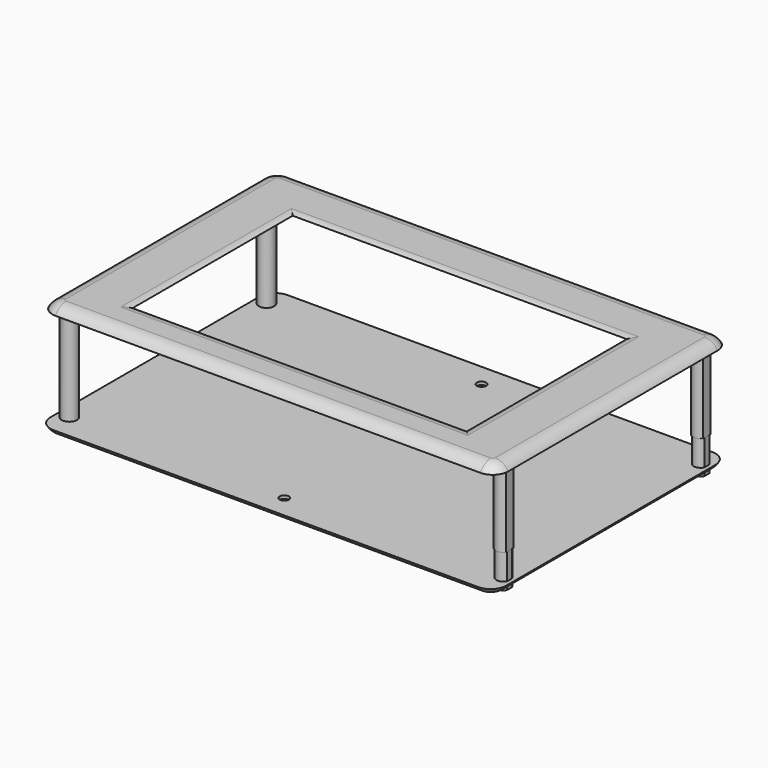
from build123d import *

# Parameters (mm, degrees)
F0_W          = 134
F0_H          = 95
F0_R          = 3
F0_W_2        = 120
F0_H_2        = 76
F0_W_3        = 116.5
F0_H_3        = 70.5
F0_W_4        = 108.5
F0_H_4        = 65
F0_R_2        = 1.5
F1_DEPTH      = 2.5
F2_DEPTH      = 2
F3_DEPTH      = 0.5
F4_T1_DEPTH   = 108.5
F4_T3_DEPTH   = 65
F4_T5_DEPTH   = 85
F4_T7_DEPTH   = 138
F4_T10_ANGLE  = 90
F4_T12_ANGLE  = 90
F4_T14_ANGLE  = 90
F4_T16_ANGLE  = 90
F4_T21_DEPTH  = 70.4491776016
F4_T25_DEPTH  = 113.9491776016
F4_T32_DEPTH  = 70.4491776016
F4_T36_DEPTH  = 113.9491776016
F4_T43_DEPTH  = 113.9491776016
F4_T47_DEPTH  = 70.4491776016
F4_T54_DEPTH  = 70.4491776016
F4_T58_DEPTH  = 113.9491776016
F5_DEPTH      = 35
F6_DEPTH      = 24
F8_R          = 2.5
F8_R_2        = 1.5
F9_DEPTH      = 2.5
F10_T1_DEPTH  = 85
F10_T3_DEPTH  = 138
F10_T6_ANGLE  = 90
F10_T8_ANGLE  = 90
F10_T10_ANGLE = 90
F10_T12_ANGLE = 90
F11_DEPTH     = 1.5
F13_R         = 1.75
F14_DEPTH     = 11


# Not quite as in the source:
# - a fillet or chamfer that OpenCascade refuses, or shapes differently, is made with other operations: its cross-section is extruded or revolved along the edge and cut away or added


with BuildPart() as f1:
    # F0 (on Top) → F1 (new body)
    with BuildSketch(Plane.XY):
        with Locations((0.2218604458, 0.5862068966)):
            Rectangle(F0_W, F0_H)
        with Locations((-57.2781395542, -41.4137931034)):
            Circle(F0_R, mode=Mode.SUBTRACT)
        with Locations((57.7218604458, -41.4137931034)):
            Circle(F0_R, mode=Mode.SUBTRACT)
        with Locations((0.2218604458, 0.0862068966)):
            Rectangle(F0_W_2, F0_H_2, mode=Mode.SUBTRACT)
        with Locations((-57.2781395542, 42.5862068966)):
            Circle(F0_R, mode=Mode.SUBTRACT)
        with Locations((57.7218604458, 42.5862068966)):
            Circle(F0_R, mode=Mode.SUBTRACT)
        with BuildLine():
            Line((-66.7781395542, -46.9137931034), (-66.7781395542, 48.0862068966))
            Line((-66.7781395542, 48.0862068966), (-68.7781395542, 48.0862068966))
            ThreePointArc((-68.7781395542, 48.0862068966), (-72.3136734602, 46.6217408025), (-73.7781395542, 43.0862068966))
            Line((-73.7781395542, 43.0862068966), (-73.7781395542, -41.9137931034))
            ThreePointArc((-73.7781395542, -41.9137931034), (-72.3136734602, -45.4493270094), (-68.7781395542, -46.9137931034))
            Line((-68.7781395542, -46.9137931034), (-66.7781395542, -46.9137931034))
        make_face()
        with BuildLine():
            ThreePointArc((-72.2781395542, -37.9473820925), (-67.7781395542, -39.4473820925), (-72.2781395542, -40.9473820925))
            Line((-72.2781395542, -40.9473820925), (-72.2781395542, -37.9473820925))
        make_face(mode=Mode.SUBTRACT)
        with BuildLine():
            ThreePointArc((-72.2781395542, 42.0910126865), (-67.7781395542, 40.5910126865), (-72.2781395542, 39.0910126865))
            Line((-72.2781395542, 39.0910126865), (-72.2781395542, 42.0910126865))
        make_face(mode=Mode.SUBTRACT)
        with BuildLine():
            Line((69.2218604458, 48.0862068966), (67.2218604458, 48.0862068966))
            Line((67.2218604458, 48.0862068966), (67.2218604458, -46.9137931034))
            Line((67.2218604458, -46.9137931034), (69.2218604458, -46.9137931034))
            ThreePointArc((69.2218604458, -46.9137931034), (72.7573943517, -45.4493270094), (74.2218604458, -41.9137931034))
            Line((74.2218604458, -41.9137931034), (74.2218604458, 43.0862068966))
            ThreePointArc((74.2218604458, 43.0862068966), (72.7573943517, 46.6217408025), (69.2218604458, 48.0862068966))
        make_face()
        with BuildLine():
            ThreePointArc((72.7218604458, -40.9469694146), (68.2218604458, -39.4469694146), (72.7218604458, -37.9469694146))
            Line((72.7218604458, -37.9469694146), (72.7218604458, -40.9469694146))
        make_face(mode=Mode.SUBTRACT)
        with BuildLine():
            ThreePointArc((72.7218604458, 39.0908259189), (68.2218604458, 40.5908259189), (72.7218604458, 42.0908259189))
            Line((72.7218604458, 42.0908259189), (72.7218604458, 39.0908259189))
        make_face(mode=Mode.SUBTRACT)
        with Locations((-57.2781395542, 42.5862068966)):
            Circle(F0_R)
        with Locations((57.7218604458, 42.5862068966)):
            Circle(F0_R)
        with Locations((57.7218604458, -41.4137931034)):
            Circle(F0_R)
        with Locations((-57.2781395542, -41.4137931034)):
            Circle(F0_R)
        with Locations((0.2218604458, 0.0862068966)):
            Rectangle(F0_W_2, F0_H_2)
        with Locations((0.4718604458, -1.1637931034)):
            Rectangle(F0_W_3, F0_H_3, mode=Mode.SUBTRACT)
        with Locations((0.4718604458, -1.1637931034)):
            Rectangle(F0_W_3, F0_H_3)
        with Locations((0.4718604458, -1.9137931034)):
            Rectangle(F0_W_4, F0_H_4, mode=Mode.SUBTRACT)
        with BuildLine():
            Line((-72.2781395542, 42.0910126865), (-72.2781395542, 39.0910126865))
            ThreePointArc((-72.2781395542, 39.0910126865), (-67.7781395542, 40.5910126865), (-72.2781395542, 42.0910126865))
        make_face()
        with Locations((-70.2781395542, 40.5910126865)):
            Circle(F0_R_2, mode=Mode.SUBTRACT)
        with Locations((-70.2781395542, 40.5910126865)):
            Circle(F0_R_2)
        with BuildLine():
            Line((-72.2781395542, -37.9473820925), (-72.2781395542, -40.9473820925))
            ThreePointArc((-72.2781395542, -40.9473820925), (-67.7781395542, -39.4473820925), (-72.2781395542, -37.9473820925))
        make_face()
        with Locations((-70.2781395542, -39.4473820925)):
            Circle(F0_R_2, mode=Mode.SUBTRACT)
        with Locations((-70.2781395542, -39.4473820925)):
            Circle(F0_R_2)
        with BuildLine():
            Line((72.7218604458, -40.9469694146), (72.7218604458, -37.9469694146))
            ThreePointArc((72.7218604458, -37.9469694146), (68.2218604458, -39.4469694146), (72.7218604458, -40.9469694146))
        make_face()
        with Locations((70.7218604458, -39.4469694146)):
            Circle(F0_R_2, mode=Mode.SUBTRACT)
        with Locations((70.7218604458, -39.4469694146)):
            Circle(F0_R_2)
        with BuildLine():
            Line((72.7218604458, 39.0908259189), (72.7218604458, 42.0908259189))
            ThreePointArc((72.7218604458, 42.0908259189), (68.2218604458, 40.5908259189), (72.7218604458, 39.0908259189))
        make_face()
        with Locations((70.7218604458, 40.5908259189)):
            Circle(F0_R_2, mode=Mode.SUBTRACT)
        with Locations((70.7218604458, 40.5908259189)):
            Circle(F0_R_2)
    extrude(amount=F1_DEPTH)

    # F0 (on Top) → F2 (cut)
    with BuildSketch(Plane.XY):
        with Locations((-57.2781395542, 42.5862068966)):
            Circle(F0_R)
        with Locations((-57.2781395542, -41.4137931034)):
            Circle(F0_R)
        with Locations((57.7218604458, -41.4137931034)):
            Circle(F0_R)
        with Locations((57.7218604458, 42.5862068966)):
            Circle(F0_R)
        with Locations((0.4718604458, -1.1637931034)):
            Rectangle(F0_W_3, F0_H_3)
        with Locations((0.4718604458, -1.9137931034)):
            Rectangle(F0_W_4, F0_H_4, mode=Mode.SUBTRACT)
    extrude(amount=F2_DEPTH, mode=Mode.SUBTRACT)

    # F0 (on Top) → F3 (cut)
    with BuildSketch(Plane.XY):
        with Locations((0.2218604458, 0.0862068966)):
            Rectangle(F0_W_2, F0_H_2)
        with Locations((0.4718604458, -1.1637931034)):
            Rectangle(F0_W_3, F0_H_3, mode=Mode.SUBTRACT)
    extrude(amount=F3_DEPTH, mode=Mode.SUBTRACT)

    # F4: fillet of radius 5 on 12 edges, made by hand

    # F4_s2 → F4_t1 (cut)
    with BuildSketch(Plane.YZ.offset(-53.7781395542)):
        with BuildLine():
            ThreePointArc((32.7658779005, 2.5004), (31.647646516, 2.3737873637), (30.5860325565, 2.0003600077))
            Line((30.5860325565, 2.0003600077), (30.3680480221, 2.450492577))
            ThreePointArc((30.3680480221, 2.450492577), (30.086070328, 2.2501800039), (30.086070328, 2.5))
            Line((30.086070328, 2.5), (30.5862068966, 3.0001365685))
            ThreePointArc((30.5862068966, 3.0001365685), (31.6760423985, 3.0001365685), (32.7658779005, 3.0005365685))
            Line((32.7658779005, 3.0005365685), (32.7658779005, 2.5004))
        make_face()
        with BuildLine():
            ThreePointArc((-36.5934641074, 2.5004), (-35.4752327229, 2.3737873637), (-34.4136187634, 2.0003600077))
            Line((-34.4136187634, 2.0003600077), (-34.195634229, 2.450492577))
            ThreePointArc((-34.195634229, 2.450492577), (-33.9136565349, 2.2501800039), (-33.9136565349, 2.5))
            Line((-33.9136565349, 2.5), (-34.4137931034, 3.0001365685))
            ThreePointArc((-34.4137931034, 3.0001365685), (-35.5036286054, 3.0001365685), (-36.5934641074, 3.0005365685))
            Line((-36.5934641074, 3.0005365685), (-36.5934641074, 2.5004))
        make_face()
    extrude(amount=F4_T1_DEPTH, mode=Mode.SUBTRACT)

    # F4_s4 → F4_t3 (cut)
    with BuildSketch(Plane.XZ.offset(-30.5862068966)):
        with BuildLine():
            ThreePointArc((-55.9578105582, 2.5004), (-54.8395791736, 2.3737873637), (-53.7779652142, 2.0003600077))
            Line((-53.7779652142, 2.0003600077), (-53.5599806798, 2.450492577))
            ThreePointArc((-53.5599806798, 2.450492577), (-53.2780029857, 2.2501800039), (-53.2780029857, 2.5))
            Line((-53.2780029857, 2.5), (-53.7781395542, 3.0001365685))
            ThreePointArc((-53.7781395542, 3.0001365685), (-54.8679750562, 3.0001365685), (-55.9578105582, 3.0005365685))
            Line((-55.9578105582, 3.0005365685), (-55.9578105582, 2.5004))
        make_face()
        with BuildLine():
            ThreePointArc((56.9015314497, 2.5004), (55.7833000652, 2.3737873637), (54.7216861058, 2.0003600077))
            Line((54.7216861058, 2.0003600077), (54.5037015714, 2.450492577))
            ThreePointArc((54.5037015714, 2.450492577), (54.2217238772, 2.2501800039), (54.2217238772, 2.5))
            Line((54.2217238772, 2.5), (54.7218604458, 3.0001365685))
            ThreePointArc((54.7218604458, 3.0001365685), (55.8116959477, 3.0001365685), (56.9015314497, 3.0005365685))
            Line((56.9015314497, 3.0005365685), (56.9015314497, 2.5004))
        make_face()
    extrude(amount=F4_T3_DEPTH, mode=Mode.SUBTRACT)

    # F4_s6 → F4_t5 (cut)
    with BuildSketch(Plane.XZ.offset(-43.0862068966)):
        with BuildLine():
            ThreePointArc((69.891175924, 2.5004), (72.3916173144, 1.8304834454), (74.2222068336, 0.0002000386))
            Line((74.2222068336, 0.0002000386), (74.6553099246, 0.250316611))
            ThreePointArc((74.6553099246, 0.250316611), (74.7219970143, 1.2501000193), (74.7219970143, 2.5))
            Line((74.7219970143, 2.5), (74.2218604458, 3.0001365685))
            ThreePointArc((74.2218604458, 3.0001365685), (72.0565181849, 3.0001365685), (69.891175924, 3.0005365685))
            Line((69.891175924, 3.0005365685), (69.891175924, 2.5004))
        make_face()
        with BuildLine():
            ThreePointArc((-73.7784859421, 0.0002000386), (-71.9478964228, 1.8304834454), (-69.4474550324, 2.5004))
            Line((-69.4474550324, 2.5004), (-69.4474550324, 3.0005365685))
            ThreePointArc((-69.4474550324, 3.0005365685), (-71.6127972933, 3.0001365685), (-73.7781395542, 3.0001365685))
            Line((-73.7781395542, 3.0001365685), (-74.2782761228, 2.5))
            ThreePointArc((-74.2782761228, 2.5), (-74.2782761228, 1.2501000193), (-74.211589033, 0.250316611))
            Line((-74.211589033, 0.250316611), (-73.7784859421, 0.0002000386))
        make_face()
    extrude(amount=F4_T5_DEPTH, mode=Mode.SUBTRACT)

    # F4_s8 → F4_t7 (cut)
    with BuildSketch(Plane.YZ.offset(-68.7781395542)):
        with BuildLine():
            ThreePointArc((48.0865532844, 0.0002000386), (46.2559637652, 1.8304834454), (43.7555223748, 2.5004))
            Line((43.7555223748, 2.5004), (43.7555223748, 3.0005365685))
            ThreePointArc((43.7555223748, 3.0005365685), (45.9208646357, 3.0001365685), (48.0862068966, 3.0001365685))
            Line((48.0862068966, 3.0001365685), (48.5863434651, 2.5))
            ThreePointArc((48.5863434651, 2.5), (48.5863434651, 1.2501000193), (48.5196563754, 0.250316611))
            Line((48.5196563754, 0.250316611), (48.0865532844, 0.0002000386))
        make_face()
        with BuildLine():
            ThreePointArc((-42.5831085817, 2.5004), (-45.0835499721, 1.8304834454), (-46.9141394913, 0.0002000386))
            Line((-46.9141394913, 0.0002000386), (-47.3472425823, 0.250316611))
            ThreePointArc((-47.3472425823, 0.250316611), (-47.413929672, 1.2501000193), (-47.413929672, 2.5))
            Line((-47.413929672, 2.5), (-46.9137931034, 3.0001365685))
            ThreePointArc((-46.9137931034, 3.0001365685), (-44.7484508426, 3.0001365685), (-42.5831085817, 3.0005365685))
            Line((-42.5831085817, 3.0005365685), (-42.5831085817, 2.5004))
        make_face()
    extrude(amount=F4_T7_DEPTH, mode=Mode.SUBTRACT)

    # F4_s9 → F4_t10 (revolve, cut)
    with BuildSketch(Plane.XZ.offset(-43.0862068966)):
        with BuildLine():
            ThreePointArc((69.891175924, 2.5004), (72.3916173144, 1.8304834454), (74.2222068336, 0.0002000386))
            Line((74.2222068336, 0.0002000386), (74.6553099246, 0.250316611))
            ThreePointArc((74.6553099246, 0.250316611), (74.7219970143, 1.2501000193), (74.7219970143, 2.5))
            Line((74.7219970143, 2.5), (74.2218604458, 3.0001365685))
            ThreePointArc((74.2218604458, 3.0001365685), (72.0565181849, 3.0001365685), (69.891175924, 3.0005365685))
            Line((69.891175924, 3.0005365685), (69.891175924, 2.5004))
        make_face()
    revolve(axis=Axis((69.2218604458, 43.0862068966, 2.5), (0, 0, 1)), revolution_arc=F4_T10_ANGLE, mode=Mode.SUBTRACT)

    # F4_s11 → F4_t12 (revolve, cut)
    with BuildSketch(Plane.YZ.offset(69.2218604458)):
        with BuildLine():
            ThreePointArc((-42.5831085817, 2.5004), (-45.0835499721, 1.8304834454), (-46.9141394913, 0.0002000386))
            Line((-46.9141394913, 0.0002000386), (-47.3472425823, 0.250316611))
            ThreePointArc((-47.3472425823, 0.250316611), (-47.413929672, 1.2501000193), (-47.413929672, 2.5))
            Line((-47.413929672, 2.5), (-46.9137931034, 3.0001365685))
            ThreePointArc((-46.9137931034, 3.0001365685), (-44.7484508426, 3.0001365685), (-42.5831085817, 3.0005365685))
            Line((-42.5831085817, 3.0005365685), (-42.5831085817, 2.5004))
        make_face()
    revolve(axis=Axis((69.2218604458, -41.9137931034, 2.5), (0, 0, 1)), revolution_arc=F4_T12_ANGLE, mode=Mode.SUBTRACT)

    # F4_s13 → F4_t14 (revolve, cut)
    with BuildSketch(Plane.XZ.offset(41.9137931034)):
        with BuildLine():
            ThreePointArc((-69.4474550324, 2.5004), (-71.9478964228, 1.8304834454), (-73.7784859421, 0.0002000386))
            Line((-73.7784859421, 0.0002000386), (-74.211589033, 0.250316611))
            ThreePointArc((-74.211589033, 0.250316611), (-74.2782761228, 1.2501000193), (-74.2782761228, 2.5))
            Line((-74.2782761228, 2.5), (-73.7781395542, 3.0001365685))
            ThreePointArc((-73.7781395542, 3.0001365685), (-71.6127972933, 3.0001365685), (-69.4474550324, 3.0005365685))
            Line((-69.4474550324, 3.0005365685), (-69.4474550324, 2.5004))
        make_face()
    revolve(axis=Axis((-68.7781395542, -41.9137931034, 2.5), (0, 0, 1)), revolution_arc=F4_T14_ANGLE, mode=Mode.SUBTRACT)

    # F4_s15 → F4_t16 (revolve, cut)
    with BuildSketch(Plane.YZ.offset(-68.7781395542)):
        with BuildLine():
            ThreePointArc((48.0865532844, 0.0002000386), (46.2559637652, 1.8304834454), (43.7555223748, 2.5004))
            Line((43.7555223748, 2.5004), (43.7555223748, 3.0005365685))
            ThreePointArc((43.7555223748, 3.0005365685), (45.9208646357, 3.0001365685), (48.0862068966, 3.0001365685))
            Line((48.0862068966, 3.0001365685), (48.5863434651, 2.5))
            ThreePointArc((48.5863434651, 2.5), (48.5863434651, 1.2501000193), (48.5196563754, 0.250316611))
            Line((48.5196563754, 0.250316611), (48.0865532844, 0.0002000386))
        make_face()
    revolve(axis=Axis((-68.7781395542, 43.0862068966, 2.5), (0, 0, 1)), revolution_arc=F4_T16_ANGLE, mode=Mode.SUBTRACT)


with BuildPart() as f4_tool19:
    # F4_s20 → F4_t21 (new body)
    with BuildSketch(Plane.XZ.offset(34.4137931034)):
        with BuildLine():
            ThreePointArc((-55.9578105582, 2.5004), (-54.8395791736, 2.3737873637), (-53.7779652142, 2.0003600077))
            Line((-53.7779652142, 2.0003600077), (-53.5599806798, 2.450492577))
            ThreePointArc((-53.5599806798, 2.450492577), (-53.2780029857, 2.2501800039), (-53.2780029857, 2.5))
            Line((-53.2780029857, 2.5), (-53.7781395542, 3.0001365685))
            ThreePointArc((-53.7781395542, 3.0001365685), (-54.8679750562, 3.0001365685), (-55.9578105582, 3.0005365685))
            Line((-55.9578105582, 3.0005365685), (-55.9578105582, 2.5004))
        make_face()
    extrude(amount=-F4_T21_DEPTH)

    split(bisect_by=Plane.XZ.offset(-30.5862068966), keep=Keep.BOTTOM)


with BuildPart() as f4_tool23:
    # F4_s24 → F4_t25 (new body)
    with BuildSketch(Plane.YZ.offset(-59.2273171558)):
        with BuildLine():
            ThreePointArc((32.7658779005, 2.5004), (31.647646516, 2.3737873637), (30.5860325565, 2.0003600077))
            Line((30.5860325565, 2.0003600077), (30.3680480221, 2.450492577))
            ThreePointArc((30.3680480221, 2.450492577), (30.086070328, 2.2501800039), (30.086070328, 2.5))
            Line((30.086070328, 2.5), (30.5862068966, 3.0001365685))
            ThreePointArc((30.5862068966, 3.0001365685), (31.6760423985, 3.0001365685), (32.7658779005, 3.0005365685))
            Line((32.7658779005, 3.0005365685), (32.7658779005, 2.5004))
        make_face()
    extrude(amount=F4_T25_DEPTH)

    split(bisect_by=Plane.YZ.offset(-53.7781395542), keep=Keep.BOTTOM)


with BuildPart() as f4_tool19_1:
    add(f4_tool19.part)

    # F4_t27: intersect F4_tool23
    add(f4_tool23.part, mode=Mode.INTERSECT)


with BuildPart() as f1_1:
    add(f1.part)

    # F4_t17: cut F4_tool19
    add(f4_tool19_1.part, mode=Mode.SUBTRACT)


with BuildPart() as f4_tool30:
    # F4_s31 → F4_t32 (new body)
    with BuildSketch(Plane.XZ.offset(-36.0353844982)):
        with BuildLine():
            ThreePointArc((56.9015314497, 2.5004), (55.7833000652, 2.3737873637), (54.7216861058, 2.0003600077))
            Line((54.7216861058, 2.0003600077), (54.5037015714, 2.450492577))
            ThreePointArc((54.5037015714, 2.450492577), (54.2217238772, 2.2501800039), (54.2217238772, 2.5))
            Line((54.2217238772, 2.5), (54.7218604458, 3.0001365685))
            ThreePointArc((54.7218604458, 3.0001365685), (55.8116959477, 3.0001365685), (56.9015314497, 3.0005365685))
            Line((56.9015314497, 3.0005365685), (56.9015314497, 2.5004))
        make_face()
    extrude(amount=F4_T32_DEPTH)

    split(bisect_by=Plane.XZ.offset(-30.5862068966), keep=Keep.BOTTOM)


with BuildPart() as f4_tool34:
    # F4_s35 → F4_t36 (new body)
    with BuildSketch(Plane.YZ.offset(-53.7781395542)):
        with BuildLine():
            ThreePointArc((32.7658779005, 2.5004), (31.647646516, 2.3737873637), (30.5860325565, 2.0003600077))
            Line((30.5860325565, 2.0003600077), (30.3680480221, 2.450492577))
            ThreePointArc((30.3680480221, 2.450492577), (30.086070328, 2.2501800039), (30.086070328, 2.5))
            Line((30.086070328, 2.5), (30.5862068966, 3.0001365685))
            ThreePointArc((30.5862068966, 3.0001365685), (31.6760423985, 3.0001365685), (32.7658779005, 3.0005365685))
            Line((32.7658779005, 3.0005365685), (32.7658779005, 2.5004))
        make_face()
    extrude(amount=F4_T36_DEPTH)

    split(bisect_by=Plane.YZ.offset(54.7218604458), keep=Keep.TOP)


with BuildPart() as f4_tool30_1:
    add(f4_tool30.part)

    # F4_t38: intersect F4_tool34
    add(f4_tool34.part, mode=Mode.INTERSECT)


with BuildPart() as f1_2:
    add(f1_1.part)

    # F4_t28: cut F4_tool30
    add(f4_tool30_1.part, mode=Mode.SUBTRACT)


with BuildPart() as f4_tool41:
    # F4_s42 → F4_t43 (new body)
    with BuildSketch(Plane.YZ.offset(54.7218604458)):
        with BuildLine():
            ThreePointArc((-36.5934641074, 2.5004), (-35.4752327229, 2.3737873637), (-34.4136187634, 2.0003600077))
            Line((-34.4136187634, 2.0003600077), (-34.195634229, 2.450492577))
            ThreePointArc((-34.195634229, 2.450492577), (-33.9136565349, 2.2501800039), (-33.9136565349, 2.5))
            Line((-33.9136565349, 2.5), (-34.4137931034, 3.0001365685))
            ThreePointArc((-34.4137931034, 3.0001365685), (-35.5036286054, 3.0001365685), (-36.5934641074, 3.0005365685))
            Line((-36.5934641074, 3.0005365685), (-36.5934641074, 2.5004))
        make_face()
    extrude(amount=-F4_T43_DEPTH)

    split(bisect_by=Plane.YZ.offset(-53.7781395542), keep=Keep.BOTTOM)


with BuildPart() as f4_tool45:
    # F4_s46 → F4_t47 (new body)
    with BuildSketch(Plane.XZ.offset(39.8629707051)):
        with BuildLine():
            ThreePointArc((-55.9578105582, 2.5004), (-54.8395791736, 2.3737873637), (-53.7779652142, 2.0003600077))
            Line((-53.7779652142, 2.0003600077), (-53.5599806798, 2.450492577))
            ThreePointArc((-53.5599806798, 2.450492577), (-53.2780029857, 2.2501800039), (-53.2780029857, 2.5))
            Line((-53.2780029857, 2.5), (-53.7781395542, 3.0001365685))
            ThreePointArc((-53.7781395542, 3.0001365685), (-54.8679750562, 3.0001365685), (-55.9578105582, 3.0005365685))
            Line((-55.9578105582, 3.0005365685), (-55.9578105582, 2.5004))
        make_face()
    extrude(amount=-F4_T47_DEPTH)

    split(bisect_by=Plane.XZ.offset(34.4137931034), keep=Keep.TOP)


with BuildPart() as f4_tool41_1:
    add(f4_tool41.part)

    # F4_t49: intersect F4_tool45
    add(f4_tool45.part, mode=Mode.INTERSECT)


with BuildPart() as f1_3:
    add(f1_2.part)

    # F4_t39: cut F4_tool41
    add(f4_tool41_1.part, mode=Mode.SUBTRACT)


with BuildPart() as f4_tool52:
    # F4_s53 → F4_t54 (new body)
    with BuildSketch(Plane.XZ.offset(-30.5862068966)):
        with BuildLine():
            ThreePointArc((56.9015314497, 2.5004), (55.7833000652, 2.3737873637), (54.7216861058, 2.0003600077))
            Line((54.7216861058, 2.0003600077), (54.5037015714, 2.450492577))
            ThreePointArc((54.5037015714, 2.450492577), (54.2217238772, 2.2501800039), (54.2217238772, 2.5))
            Line((54.2217238772, 2.5), (54.7218604458, 3.0001365685))
            ThreePointArc((54.7218604458, 3.0001365685), (55.8116959477, 3.0001365685), (56.9015314497, 3.0005365685))
            Line((56.9015314497, 3.0005365685), (56.9015314497, 2.5004))
        make_face()
    extrude(amount=F4_T54_DEPTH)

    split(bisect_by=Plane.XZ.offset(34.4137931034), keep=Keep.TOP)


with BuildPart() as f4_tool56:
    # F4_s57 → F4_t58 (new body)
    with BuildSketch(Plane.YZ.offset(60.1710380474)):
        with BuildLine():
            ThreePointArc((-36.5934641074, 2.5004), (-35.4752327229, 2.3737873637), (-34.4136187634, 2.0003600077))
            Line((-34.4136187634, 2.0003600077), (-34.195634229, 2.450492577))
            ThreePointArc((-34.195634229, 2.450492577), (-33.9136565349, 2.2501800039), (-33.9136565349, 2.5))
            Line((-33.9136565349, 2.5), (-34.4137931034, 3.0001365685))
            ThreePointArc((-34.4137931034, 3.0001365685), (-35.5036286054, 3.0001365685), (-36.5934641074, 3.0005365685))
            Line((-36.5934641074, 3.0005365685), (-36.5934641074, 2.5004))
        make_face()
    extrude(amount=-F4_T58_DEPTH)

    split(bisect_by=Plane.YZ.offset(54.7218604458), keep=Keep.TOP)


with BuildPart() as f4_tool52_1:
    add(f4_tool52.part)

    # F4_t60: intersect F4_tool56
    add(f4_tool56.part, mode=Mode.INTERSECT)


with BuildPart() as f1_4:
    add(f1_3.part)

    # F4_t50: cut F4_tool52
    add(f4_tool52_1.part, mode=Mode.SUBTRACT)

    # F0 (on Top) → F5 (join)
    with BuildSketch(Plane.XY):
        with BuildLine():
            Line((-72.2781395542, 42.0910126865), (-72.2781395542, 39.0910126865))
            ThreePointArc((-72.2781395542, 39.0910126865), (-67.7781395542, 40.5910126865), (-72.2781395542, 42.0910126865))
        make_face()
        with Locations((-70.2781395542, 40.5910126865)):
            Circle(F0_R_2, mode=Mode.SUBTRACT)
        with BuildLine():
            Line((-72.2781395542, -37.9473820925), (-72.2781395542, -40.9473820925))
            ThreePointArc((-72.2781395542, -40.9473820925), (-67.7781395542, -39.4473820925), (-72.2781395542, -37.9473820925))
        make_face()
        with Locations((-70.2781395542, -39.4473820925)):
            Circle(F0_R_2, mode=Mode.SUBTRACT)
    extrude(amount=-F5_DEPTH)

    # F0 (on Top) → F6 (join)
    with BuildSketch(Plane.XY):
        with BuildLine():
            Line((72.7218604458, 39.0908259189), (72.7218604458, 42.0908259189))
            ThreePointArc((72.7218604458, 42.0908259189), (68.2218604458, 40.5908259189), (72.7218604458, 39.0908259189))
        make_face()
        with Locations((70.7218604458, 40.5908259189)):
            Circle(F0_R_2, mode=Mode.SUBTRACT)
        with BuildLine():
            Line((72.7218604458, -40.9469694146), (72.7218604458, -37.9469694146))
            ThreePointArc((72.7218604458, -37.9469694146), (68.2218604458, -39.4469694146), (72.7218604458, -40.9469694146))
        make_face()
        with Locations((70.7218604458, -39.4469694146)):
            Circle(F0_R_2, mode=Mode.SUBTRACT)
    extrude(amount=-F6_DEPTH)

    # F13 (on offset) → F14 (join)
    with BuildSketch(Plane.XY.offset(-24)):
        with BuildLine():
            Line((72.6938952208, 39.580498134), (72.6938952208, 41.6420509468))
            ThreePointArc((72.6938952208, 41.6420509468), (68.4438952208, 40.6112745404), (72.6938952208, 39.580498134))
        make_face()
        with Locations((70.6938952208, 40.6112745404)):
            Circle(F13_R, mode=Mode.SUBTRACT)
        with BuildLine():
            Line((72.6938952208, -40.4877920996), (72.6938952208, -38.4262392868))
            ThreePointArc((72.6938952208, -38.4262392868), (68.4438952208, -39.4570156932), (72.6938952208, -40.4877920996))
        make_face()
        with Locations((70.6938952208, -39.4570156932)):
            Circle(F13_R, mode=Mode.SUBTRACT)
    extrude(amount=-F14_DEPTH)


with BuildPart() as f9:
    # F8 (on offset) → F9 (new body)
    with BuildSketch(Plane.XY.offset(-35)):
        with BuildLine():
            ThreePointArc((-74, -42.5), (-72.5355339059, -46.0355339059), (-69, -47.5))
            Line((-69, -47.5), (69, -47.5))
            ThreePointArc((69, -47.5), (72.5355339059, -46.0355339059), (74, -42.5))
            Line((74, -42.5), (74, 42.5))
            ThreePointArc((74, 42.5), (72.5355339059, 46.0355339059), (69, 47.5))
            Line((69, 47.5), (-69, 47.5))
            ThreePointArc((-69, 47.5), (-72.5355339059, 46.0355339059), (-74, 42.5))
            Line((-74, 42.5), (-74, -42.5))
        make_face()
        with Locations((-70.5, -40.03359)):
            Circle(F8_R, mode=Mode.SUBTRACT)
        with Locations((0, -40.03359)):
            Circle(F8_R, mode=Mode.SUBTRACT)
        with Locations((70.5, -40.03318)):
            Circle(F8_R, mode=Mode.SUBTRACT)
        with Locations((-70.5, 40.00481)):
            Circle(F8_R, mode=Mode.SUBTRACT)
        with Locations((0, 40.00481)):
            Circle(F8_R, mode=Mode.SUBTRACT)
        with Locations((70.5, 40.00462)):
            Circle(F8_R, mode=Mode.SUBTRACT)
        with Locations((-70.5, 40.00481)):
            Circle(F8_R)
        with Locations((-70.5, 40.00481)):
            Circle(F8_R_2, mode=Mode.SUBTRACT)
        with Locations((-70.5, -40.03359)):
            Circle(F8_R)
        with Locations((-70.5, -40.03359)):
            Circle(F8_R_2, mode=Mode.SUBTRACT)
        with Locations((0, 40.00481)):
            Circle(F8_R)
        with Locations((0, 40.00481)):
            Circle(F8_R_2, mode=Mode.SUBTRACT)
        with Locations((0, -40.03359)):
            Circle(F8_R)
        with Locations((0, -40.03359)):
            Circle(F8_R_2, mode=Mode.SUBTRACT)
        with Locations((70.5, 40.00462)):
            Circle(F8_R)
        with Locations((70.5, 40.00462)):
            Circle(F8_R_2, mode=Mode.SUBTRACT)
        with Locations((70.5, -40.03318)):
            Circle(F8_R)
        with Locations((70.5, -40.03318)):
            Circle(F8_R_2, mode=Mode.SUBTRACT)
    extrude(amount=F9_DEPTH)

    # F10: fillet of radius 5 on 1 edges, made by hand

    # F10_s2 → F10_t1 (cut)
    with BuildSketch(Plane.XZ.offset(-42.5)):
        with BuildLine():
            ThreePointArc((-74, -32.5), (-72.1698729811, -34.3301270189), (-69.6698729811, -35))
            Line((-69.6698729811, -35), (-74, -35))
            Line((-74, -35), (-74, -32.5))
        make_face()
        with BuildLine():
            ThreePointArc((74, -32.5), (72.1698729811, -34.3301270189), (69.6698729811, -35))
            Line((69.6698729811, -35), (74, -35))
            Line((74, -35), (74, -32.5))
        make_face()
    extrude(amount=F10_T1_DEPTH, mode=Mode.SUBTRACT)

    # F10_s4 → F10_t3 (cut)
    with BuildSketch(Plane.YZ.offset(-69)):
        with BuildLine():
            ThreePointArc((-47.5, -32.5), (-45.6698729811, -34.3301270189), (-43.1698729811, -35))
            Line((-43.1698729811, -35), (-47.5, -35))
            Line((-47.5, -35), (-47.5, -32.5))
        make_face()
        with BuildLine():
            ThreePointArc((47.5, -32.5), (45.6698729811, -34.3301270189), (43.1698729811, -35))
            Line((43.1698729811, -35), (47.5, -35))
            Line((47.5, -35), (47.5, -32.5))
        make_face()
    extrude(amount=F10_T3_DEPTH, mode=Mode.SUBTRACT)

    # F10_s5 → F10_t6 (revolve, cut)
    with BuildSketch(Plane.YZ.offset(-69)):
        with BuildLine():
            ThreePointArc((47.5, -32.5), (45.6698729811, -34.3301270189), (43.1698729811, -35))
            Line((43.1698729811, -35), (47.5, -35))
            Line((47.5, -35), (47.5, -32.5))
        make_face()
    revolve(axis=Axis((-69, 42.5, -35), (0, 0, 1)), revolution_arc=F10_T6_ANGLE, mode=Mode.SUBTRACT)

    # F10_s7 → F10_t8 (revolve, cut)
    with BuildSketch(Plane.XZ.offset(42.5)):
        with BuildLine():
            ThreePointArc((-74, -32.5), (-72.1698729811, -34.3301270189), (-69.6698729811, -35))
            Line((-69.6698729811, -35), (-74, -35))
            Line((-74, -35), (-74, -32.5))
        make_face()
    revolve(axis=Axis((-69, -42.5, -35), (0, 0, 1)), revolution_arc=F10_T8_ANGLE, mode=Mode.SUBTRACT)

    # F10_s9 → F10_t10 (revolve, cut)
    with BuildSketch(Plane.YZ.offset(69)):
        with BuildLine():
            ThreePointArc((-47.5, -32.5), (-45.6698729811, -34.3301270189), (-43.1698729811, -35))
            Line((-43.1698729811, -35), (-47.5, -35))
            Line((-47.5, -35), (-47.5, -32.5))
        make_face()
    revolve(axis=Axis((69, -42.5, -35), (0, 0, 1)), revolution_arc=F10_T10_ANGLE, mode=Mode.SUBTRACT)

    # F10_s11 → F10_t12 (revolve, cut)
    with BuildSketch(Plane.XZ.offset(-42.5)):
        with BuildLine():
            ThreePointArc((74, -32.5), (72.1698729811, -34.3301270189), (69.6698729811, -35))
            Line((69.6698729811, -35), (74, -35))
            Line((74, -35), (74, -32.5))
        make_face()
    revolve(axis=Axis((69, 42.5, -35), (0, 0, 1)), revolution_arc=F10_T12_ANGLE, mode=Mode.SUBTRACT)

    # F8 (on offset) → F11 (cut)
    with BuildSketch(Plane.XY.offset(-35)):
        with Locations((-70.5, 40.00481)):
            Circle(F8_R)
        with Locations((-70.5, 40.00481)):
            Circle(F8_R_2, mode=Mode.SUBTRACT)
        with Locations((-70.5, -40.03359)):
            Circle(F8_R)
        with Locations((-70.5, -40.03359)):
            Circle(F8_R_2, mode=Mode.SUBTRACT)
        with Locations((0, -40.03359)):
            Circle(F8_R)
        with Locations((0, -40.03359)):
            Circle(F8_R_2, mode=Mode.SUBTRACT)
        with Locations((0, 40.00481)):
            Circle(F8_R)
        with Locations((0, 40.00481)):
            Circle(F8_R_2, mode=Mode.SUBTRACT)
        with Locations((70.5, 40.00462)):
            Circle(F8_R)
        with Locations((70.5, 40.00462)):
            Circle(F8_R_2, mode=Mode.SUBTRACT)
        with Locations((70.5, -40.03318)):
            Circle(F8_R)
        with Locations((70.5, -40.03318)):
            Circle(F8_R_2, mode=Mode.SUBTRACT)
    extrude(amount=F11_DEPTH, mode=Mode.SUBTRACT)


solid = Compound([f1_4.part, f9.part])
